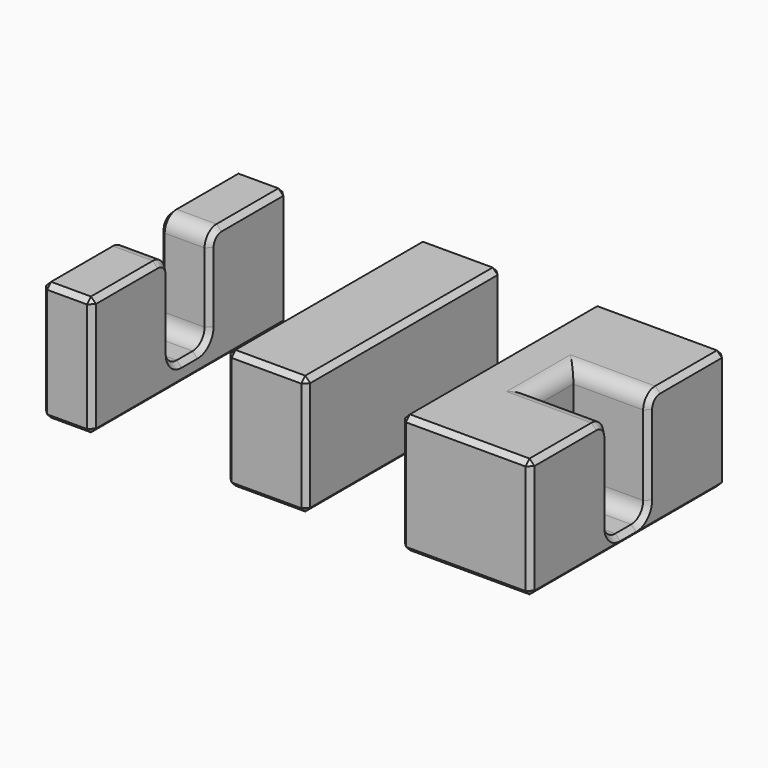
from build123d import *

# Parameters (mm, degrees)
F0_W       = 16
F0_H       = 49
F1_DEPTH   = 24
F2_SIZE    = 1
F0_W_2     = 26
F3_DEPTH   = 24
F5_DEPTH   = 15
F0_W_3     = 10
F6_DEPTH   = 24
F8_DEPTH   = 26
F9_R       = 3
F9_2_R     = 3
F10_SIZE   = 0.99999
F10_2_SIZE = 0.99999


# Not quite as in the source:
# - a fillet or chamfer is up to 0.001 mm smaller than in the source, because OpenCascade refuses the exact size


with BuildPart() as f1:
    # F0 (on Top) → F1 (new body)
    with BuildSketch(Plane.XY):
        Rectangle(F0_W, F0_H)
    extrude(amount=F1_DEPTH)

    # F2
    f2_edges = [f1.edges().sort_by_distance(p)[0] for p in [
        (-8, 0, 0),
        (0, -24.5, 0),
        (8, 0, 0),
        (0, 24.5, 0),
        (8, -24.5, 12),
        (8, 24.5, 12),
        (-8, 24.5, 12),
        (-8, -24.5, 12),
        (-8, 0, 24),
        (0, -24.5, 24),
        (8, 0, 24),
        (0, 24.5, 24),
    ]]
    chamfer(f2_edges, length=F2_SIZE)


with BuildPart() as f3:
    # F0 (on Top) → F3 (new body)
    with BuildSketch(Plane.XY):
        with Locations((40, 0)):
            Rectangle(F0_W_2, F0_H)
    extrude(amount=F3_DEPTH)

    # F4 (on face) → F5 (cut)
    with BuildSketch(Plane.YZ.offset(53)):
        Polygon((-5, 2), (0, 2), (5, 2), (5, 24), (-5, 24), align=None)
    extrude(amount=-F5_DEPTH, mode=Mode.SUBTRACT)

    # F9
    f9_edges = [f3.edges().sort_by_distance(p)[0] for p in [
        (45.5, 5, 2),
        (45.5, -5, 2),
        (38, 0, 2),
        (45.5, 5, 24),
        (38, 0, 24),
        (45.5, -5, 24),
    ]]
    fillet(f9_edges, radius=F9_R)

    # F10 (size 1 in the source; OpenCascade refuses exactly that, so slightly less here)
    f10_edges = [f3.edges().sort_by_distance(p)[0] for p in [
        (53, 16.25, 24),
        (53, 5.87868, 23.12132),
        (53, 24.5, 12),
        (53, 5, 13),
        (53, 0, 0),
        (53, 4.12132, 2.87868),
        (53, -24.5, 12),
        (53, 0, 2),
        (53, -16.25, 24),
        (53, -4.12132, 2.87868),
        (53, -5.87868, 23.12132),
        (53, -5, 13),
        (27, -24.5, 12),
        (40, -24.5, 0),
        (40, -24.5, 24),
        (27, 24.5, 12),
        (27, 0, 0),
        (27, 0, 24),
        (40, 24.5, 0),
        (40, 24.5, 24),
    ]]
    chamfer(f10_edges, length=F10_SIZE)


with BuildPart() as f6:
    # F0 (on Top) → F6 (new body)
    with BuildSketch(Plane.XY):
        with Locations((-40, 0)):
            Rectangle(F0_W_3, F0_H)
    extrude(amount=F6_DEPTH)

    # F7 (on face) → F8 (cut)
    with BuildSketch(Plane(origin=(-45, 0, 0), x_dir=(0, -1, 0), z_dir=(-1, 0, 0))):
        Polygon((-5, 4), (0, 4), (5, 4), (5, 24), (-5, 24), align=None)
    extrude(amount=-F8_DEPTH, mode=Mode.SUBTRACT)

    # F9#2
    f9_2_edges = [f6.edges().sort_by_distance(p)[0] for p in [
        (-40, -5, 4),
        (-40, 5, 4),
        (-40, 5, 24),
        (-40, -5, 24),
    ]]
    fillet(f9_2_edges, radius=F9_2_R)

    # F10#2 (size 1 in the source; OpenCascade refuses exactly that, so slightly less here)
    f10_2_edges = [f6.edges().sort_by_distance(p)[0] for p in [
        (-45, -16.25, 24),
        (-45, -5.87868, 23.12132),
        (-45, -24.5, 12),
        (-45, -5, 14),
        (-45, 0, 0),
        (-45, -4.12132, 4.87868),
        (-45, 24.5, 12),
        (-45, 0, 4),
        (-45, 16.25, 24),
        (-45, 4.12132, 4.87868),
        (-45, 5.87868, 23.12132),
        (-45, 5, 14),
        (-35, 16.25, 24),
        (-35, 5.87868, 23.12132),
        (-35, 24.5, 12),
        (-35, 5, 14),
        (-35, 0, 0),
        (-35, 4.12132, 4.87868),
        (-35, -24.5, 12),
        (-35, 0, 4),
        (-35, -16.25, 24),
        (-35, -4.12132, 4.87868),
        (-35, -5.87868, 23.12132),
        (-35, -5, 14),
        (-40, -24.5, 0),
        (-40, 24.5, 0),
        (-40, 24.5, 24),
        (-40, -24.5, 24),
    ]]
    chamfer(f10_2_edges, length=F10_2_SIZE)


solid = Compound([f1.part, f3.part, f6.part])
